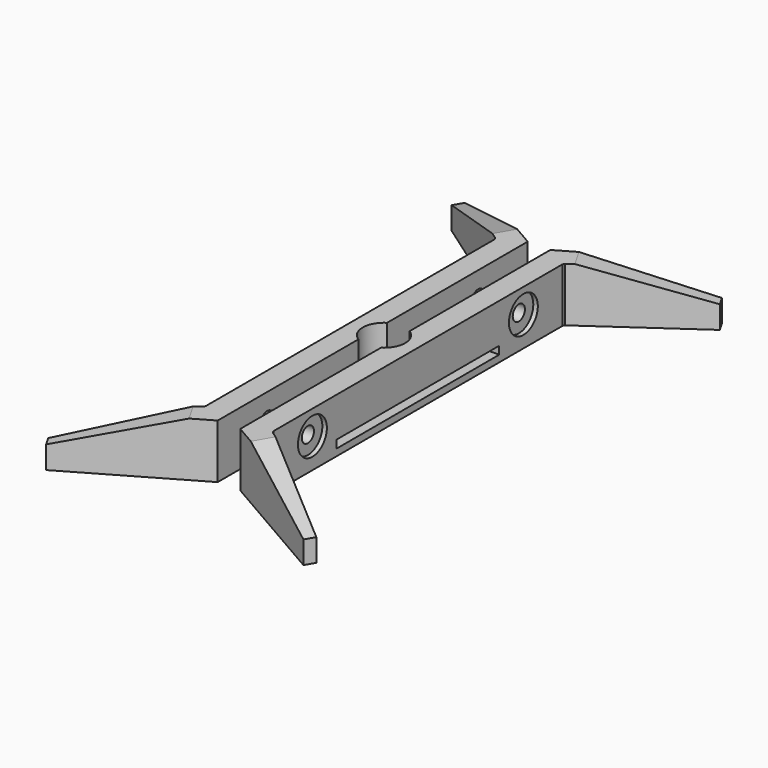
from build123d import *

# Parameters (mm, degrees)
F4_DEPTH    = 24
F5_W        = 90
F5_H        = 3.5
F5_R        = 3.375
F6_DEPTH    = 76.9625242271
F7_DEPTH    = 5
F8_R        = 8
F8_R_2      = 3.375
F9_DEPTH    = 2
F10_SIZE2   = 14
F10_SIZE    = 50
F10_2_SIZE2 = 14
F10_2_SIZE  = 50
F11_ANGLE   = 5
F12_ANGLE   = 5
F13_ANGLE   = 5
F14_ANGLE   = 5


# Not quite as in the source:
# - a feature of the source that left no trace in its solid (it failed there, or was rolled back) is left out


with BuildPart() as f4:
    # F3 (on Top) → F4 (new body)
    with BuildSketch(Plane.XY):
        Polygon((-61.9615242271, 107.1132486541), (-15, 80), (-5, 80), (-5, 85.7735026919), (-56.9615242271, 115.7735026919), align=None)
        with BuildLine():
            Line((-15, 80), (-15, -80))
            Line((-15, -80), (-5, -80))
            Line((-5, -80), (-5, -7.9303609628))
            ThreePointArc((-5, -7.9303609628), (-9.375, 0), (-5, 7.9303609628))
            Line((-5, 7.9303609628), (-5, 80))
            Line((-5, 80), (-15, 80))
        make_face()
        Polygon((-5, -80), (-15, -80), (-61.9615242271, -107.1132486541), (-56.9615242271, -115.7735026919), (-5, -85.7735026919), align=None)
    extrude(amount=F4_DEPTH)


with BuildPart() as f4b:
    # F3 (on Top) → F4, piece 2 (new body)
    with BuildSketch(Plane.XY):
        Polygon((15, -80), (5, -80), (5, -85.7735026919), (56.9615242271, -115.7735026919), (61.9615242271, -107.1132486541), align=None)
        with BuildLine():
            ThreePointArc((9.375, 0), (8.2087034604, -4.5285552332), (5, -7.9303609628))
            Line((5, -7.9303609628), (5, -80))
            Line((5, -80), (15, -80))
            Line((15, -80), (15, 80))
            Line((15, 80), (5, 80))
            Line((5, 80), (5, 7.9303609628))
            ThreePointArc((5, 7.9303609628), (8.2087034604, 4.5285552332), (9.375, 0))
        make_face()
        Polygon((5, 85.7735026919), (5, 80), (15, 80), (61.9615242271, 107.1132486541), (56.9615242271, 115.7735026919), align=None)
    extrude(amount=F4_DEPTH)


with BuildPart() as f6_tool:
    # F5 (on face) → F6 (new body, through all)
    with BuildSketch(Plane(origin=(-15, 0, 0), x_dir=(0, -1, 0), z_dir=(-1, 0, 0))):
        with Locations((0, 4.75)):
            Rectangle(F5_W, F5_H)
        with Locations((-58.3604719043, 13.25)):
            Circle(F5_R)
        with Locations((58.3604719043, 13.25)):
            Circle(F5_R)
    extrude(amount=-F6_DEPTH)


with BuildPart() as f4_1:
    add(f4.part)

    # F6: cut by f6_tool
    add(f6_tool.part, mode=Mode.SUBTRACT)

    # F5 (on face) → F7 (cut)
    with BuildSketch(Plane(origin=(-15, 0, 0), x_dir=(0, -1, 0), z_dir=(-1, 0, 0))):
        Polygon((65, 13.25), (61.6802359522, 19), (55.0407078565, 19), (51.7209438086, 13.25), (55.0407078565, 7.5), (61.6802359522, 7.5), align=None)
        with Locations((58.3604719043, 13.25)):
            Circle(F5_R, mode=Mode.SUBTRACT)
        Polygon((-51.7209438086, 13.25), (-55.0407078565, 19), (-61.6802359522, 19), (-65, 13.25), (-61.6802359522, 7.5), (-55.0407078565, 7.5), align=None)
        with Locations((-58.3604719043, 13.25)):
            Circle(F5_R, mode=Mode.SUBTRACT)
    extrude(amount=-F7_DEPTH, mode=Mode.SUBTRACT)

    # F10
    f10_edges = [f4_1.edges().sort_by_distance(p)[0] for p in [
        (-59.461524, -111.443376, 24),
        (-59.461524, 111.443376, 24),
    ]]
    f10_side = f4_1.faces().sort_by_distance((-37.28851, 95.621666, 24))[0]
    chamfer(f10_edges, length=F10_SIZE, length2=F10_SIZE2, reference=f10_side)

    # F4_face2 (on face) → F11 (revolve, cut)
    with BuildSketch(Plane(origin=(-35.1526852914, 91.6351582779, 9.3023231821), x_dir=(0.8660254038, -0.5, 0), z_dir=(-0.5, -0.8660254038, 0))):
        Polygon((-30.9561807523, 0.6976768179), (-30.9561807523, -9.3023231821), (23.2703165558, -9.3023231821), (23.2703165558, 14.6976768179), (19.0438192477, 14.6976768179), align=None)
    revolve(axis=Axis((-5, 85.7735026919, 12), (0, 0, -1)), revolution_arc=F11_ANGLE, mode=Mode.SUBTRACT)

    # F4_face5 (on face) → F14 (revolve, cut)
    with BuildSketch(Plane(origin=(-35.1526852914, -91.6351582779, 9.3023231821), x_dir=(-0.8660254038, -0.5, 0), z_dir=(-0.5, 0.8660254038, 0))):
        Polygon((30.9561807523, -9.3023231821), (30.9561807523, 0.6976768179), (-19.0438192477, 14.6976768179), (-23.2703165558, 14.6976768179), (-23.2703165558, -9.3023231821), align=None)
    revolve(axis=Axis((-5, -85.7735026919, 12), (0, 0, 1)), revolution_arc=F14_ANGLE, mode=Mode.SUBTRACT)


with BuildPart() as f4b_1:
    add(f4b.part)

    # F6: cut by f6_tool
    add(f6_tool.part, mode=Mode.SUBTRACT)

    # F8 (on face) → F9 (cut)
    with BuildSketch(Plane.YZ.offset(15)):
        with Locations((-58.3604719043, 13.25)):
            Circle(F8_R)
        with Locations((-58.3604719043, 13.25)):
            Circle(F8_R_2, mode=Mode.SUBTRACT)
        with Locations((58.3604719043, 13.25)):
            Circle(F8_R)
        with Locations((58.3604719043, 13.25)):
            Circle(F8_R_2, mode=Mode.SUBTRACT)
    extrude(amount=-F9_DEPTH, mode=Mode.SUBTRACT)

    # F10#2
    f10_2_edges = [f4b_1.edges().sort_by_distance(p)[0] for p in [
        (59.461524, 111.443376, 24),
        (59.461524, -111.443376, 24),
    ]]
    f10_2_side = f4b_1.faces().sort_by_distance((37.28851, -95.621666, 24))[0]
    chamfer(f10_2_edges, length=F10_2_SIZE, length2=F10_2_SIZE2, reference=f10_2_side)

    # F4_face3 (on face) → F12 (revolve, cut)
    with BuildSketch(Plane(origin=(35.1526852914, 91.6351582779, 9.3023231821), x_dir=(0.8660254038, 0.5, 0), z_dir=(0.5, -0.8660254038, 0))):
        Polygon((30.9561807523, -9.3023231821), (30.9561807523, 0.6976768179), (-19.0438192477, 14.6976768179), (-23.2703165558, 14.6976768179), (-23.2703165558, -9.3023231821), align=None)
    revolve(axis=Axis((5, 85.7735026919, 12), (0, 0, 1)), revolution_arc=F12_ANGLE, mode=Mode.SUBTRACT)

    # F4_face4 (on face) → F13 (revolve, cut)
    with BuildSketch(Plane(origin=(35.1526852914, -91.6351582779, 9.3023231821), x_dir=(-0.8660254038, 0.5, 0), z_dir=(0.5, 0.8660254038, 0))):
        Polygon((-30.9561807523, 0.6976768179), (-30.9561807523, -9.3023231821), (23.2703165558, -9.3023231821), (23.2703165558, 14.6976768179), (19.0438192477, 14.6976768179), align=None)
    revolve(axis=Axis((5, -85.7735026919, 12), (0, 0, -1)), revolution_arc=F13_ANGLE, mode=Mode.SUBTRACT)


solid = Compound([f4_1.part, f4b_1.part])
